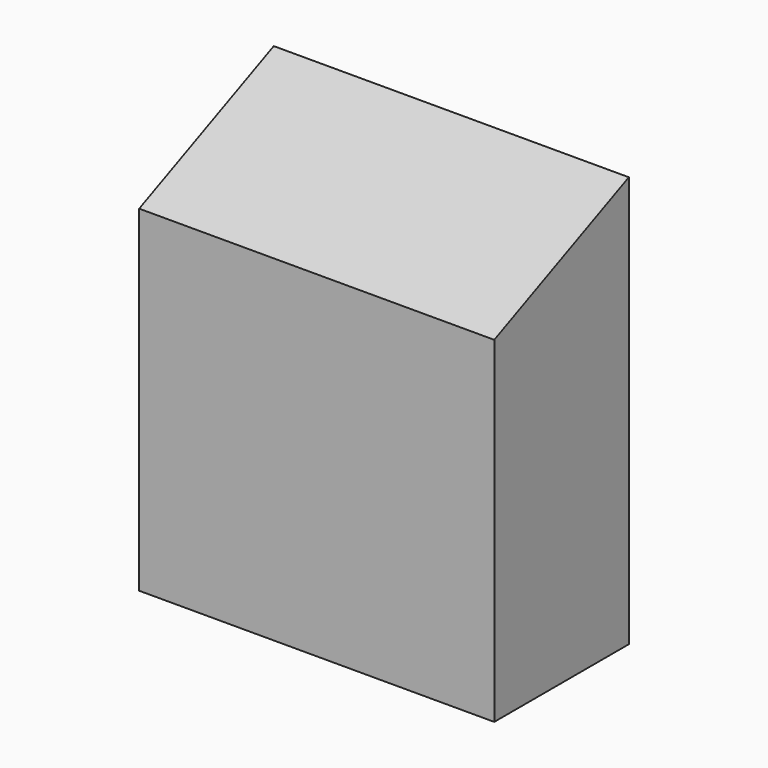
from build123d import *

# Parameters (mm, degrees)
F0_W     = 228.6
F0_H     = 558.8
F1_DEPTH = 482.6
F2_SIZE2 = 101.59999
F2_SIZE  = 228.59999


# Not quite as in the source:
# - a fillet or chamfer is up to 0.001 mm smaller than in the source, because OpenCascade refuses the exact size


with BuildPart() as f1:
    # F0 (on Right) → F1 (new body)
    with BuildSketch(Plane.YZ):
        with Locations((114.3, 279.4)):
            Rectangle(F0_W, F0_H)
    extrude(amount=-F1_DEPTH)

    # F2 (size 228.6 and 101.6 in the source; OpenCascade refuses exactly that, so slightly less here)
    f2_edges = [f1.edges().sort_by_distance(p)[0] for p in [
        (-241.3, 0, 558.8),
    ]]
    f2_side = f1.faces().sort_by_distance((-241.3, 114.3, 558.8))[0]
    chamfer(f2_edges, length=F2_SIZE, length2=F2_SIZE2, reference=f2_side)


solid = f1.part
